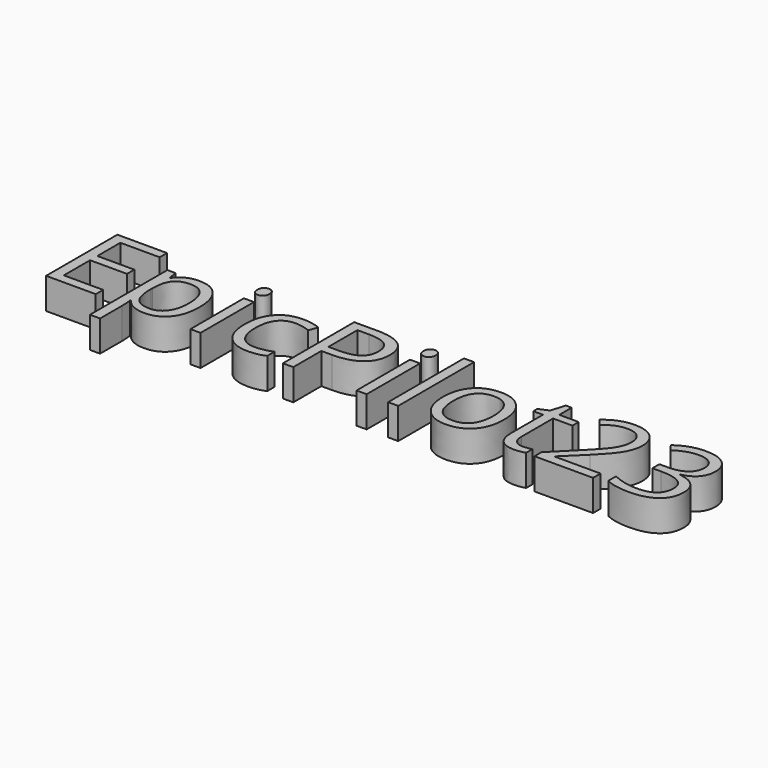
from build123d import *

# Parameters (mm, degrees)
F0_TEXT_SIZE = 102.2025580621
F1_DEPTH     = 25.4


# Not quite as in the source:
# - Text() gives the source's letters only with a copy of the font that has no kerning and outlines rounded to 1/6400 em; it was checked with that copy


with BuildPart() as f1:
    # F0 (on Top) → F1 (new body)
    with BuildSketch(Plane.XY):
        with Locations((-63.5602548718, -27.5460220873)):
            Text('EpicPilot23', F0_TEXT_SIZE, font='Open Sans', text_align=(TextAlign.LEFT, TextAlign.BOTTOM))
    extrude(amount=F1_DEPTH)


solid = f1.part
